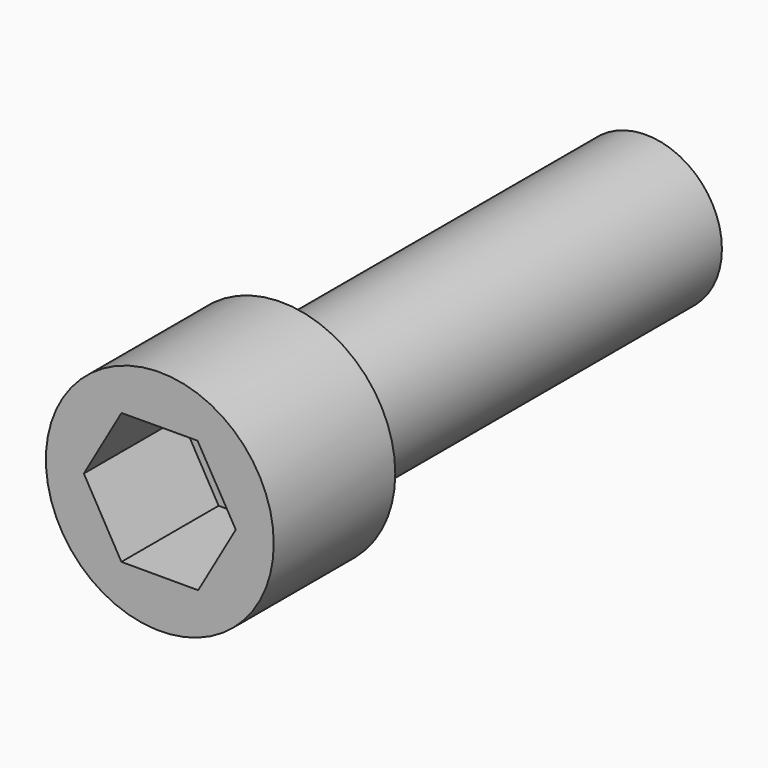
from build123d import *

# Parameters (mm, degrees)
F0_R     = 5
F1_DEPTH = 30
F3_R     = 7.5
F4_DEPTH = 10
F7_DEPTH = 8


# Not quite as in the source:
# - a feature names something its author has since deleted; it is built from what else it names


with BuildPart() as f1:
    # F0 (on Front) → F1 (new body)
    with BuildSketch(Plane.XZ):
        Circle(F0_R)
    extrude(amount=-F1_DEPTH)

    # F3 (on offset) → F4 (join)
    with BuildSketch(Plane.XZ):
        Circle(F3_R)
    extrude(amount=F4_DEPTH)

    # F6 (on offset) → F7 (cut)
    with BuildSketch(Plane.XZ.offset(10)):
        Polygon((5, 0), (2.4813610619, 4.3408348599), (-2.5225813199, 4.3170109433), (-5, 0), (-2.5277935483, -4.313961031), (2.5273847237, -4.3142005584), align=None)
    extrude(amount=-F7_DEPTH, mode=Mode.SUBTRACT)


solid = f1.part
